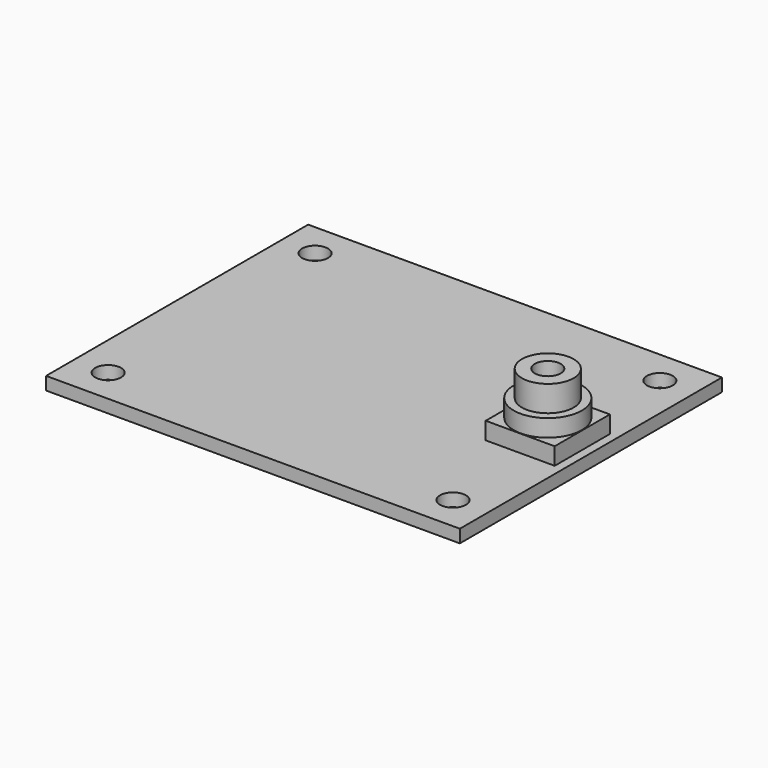
from build123d import *

# Parameters (mm, degrees)
F0_W     = 48
F0_H     = 38
F0_R     = 1.5
F1_DEPTH = 1.5
F2_R     = 3.95
F3_DEPTH = 2
F2_R_2   = 3
F4_DEPTH = 4
F2_R_3   = 1.5
F5_DEPTH = 7


with BuildPart() as f1:
    # F0 (on Top) → F1 (new body)
    with BuildSketch(Plane.XY):
        with Locations((24, 19)):
            Rectangle(F0_W, F0_H)
        with Locations((4, 4)):
            Circle(F0_R, mode=Mode.SUBTRACT)
        with Locations((44, 4)):
            Circle(F0_R, mode=Mode.SUBTRACT)
        with Locations((4, 34)):
            Circle(F0_R, mode=Mode.SUBTRACT)
        with Locations((44, 34)):
            Circle(F0_R, mode=Mode.SUBTRACT)
    extrude(amount=F1_DEPTH)


with BuildPart() as f3:
    # F2 (on face) → F3 (new body)
    with BuildSketch(Plane.XY.offset(1.5)):
        Polygon((47, 15), (47, 19), (47, 23), (39, 23), (39, 15), align=None)
        with Locations((43, 19)):
            Circle(F2_R, mode=Mode.SUBTRACT)
    extrude(amount=F3_DEPTH)

    # F2 (on face) → F4 (join)
    with BuildSketch(Plane.XY.offset(1.5)):
        with Locations((43, 19)):
            Circle(F2_R)
        with Locations((43, 19)):
            Circle(F2_R_2, mode=Mode.SUBTRACT)
    extrude(amount=F4_DEPTH)

    # F2 (on face) → F5 (join)
    with BuildSketch(Plane.XY.offset(1.5)):
        with Locations((43, 19)):
            Circle(F2_R_2)
        with Locations((43, 19)):
            Circle(F2_R_3, mode=Mode.SUBTRACT)
    extrude(amount=F5_DEPTH)


solid = Compound([f1.part, f3.part])
